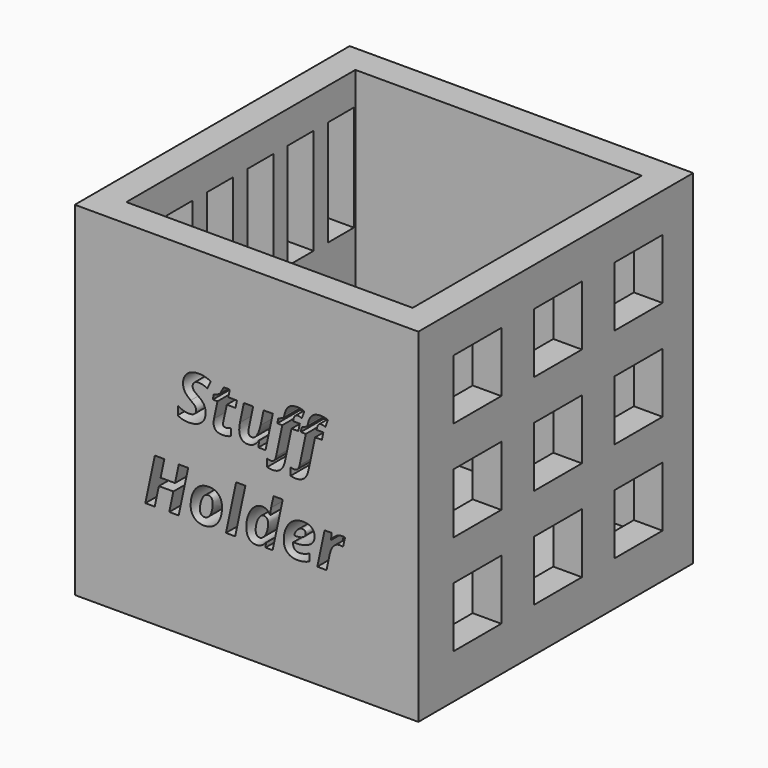
from build123d import *

# Parameters (mm, degrees)
F0_W         = 60
F0_H         = 60
F1_DEPTH     = 60
F2_W         = 50
F2_H         = 50
F3_DEPTH     = 55
F4_TEXT_SIZE = 11.0161878789
F5_DEPTH     = 10
F6_W         = 10.4811163619
F6_H         = 10.4811154306
F7_DEPTH     = 10
F8_W         = 5.6469417632
F8_H         = 18.4732027113
F9_DEPTH     = 10


# Not quite as in the source:
# - Text() gives the source's letters only with a copy of the font that has no kerning and outlines rounded to 1/6400 em; it was checked with that copy


with BuildPart() as f1:
    # F0 (on Right) → F1 (new body)
    with BuildSketch(Plane.YZ):
        with Locations((0.1416392624, -0.4152884824)):
            Rectangle(F0_W, F0_H)
    extrude(amount=F1_DEPTH)

    # F2 (on face) → F3 (cut)
    with BuildSketch(Plane.XY.offset(29.5847115176)):
        with Locations((30, 0.1416392624)):
            Rectangle(F2_W, F2_H)
    extrude(amount=-F3_DEPTH, mode=Mode.SUBTRACT)

    # F4 (on face) → F5 (cut)
    with BuildSketch(Plane.XZ.offset(29.8583607376)):
        with Locations((17.7640982414, 2.6910963934)):
            Text('Stuff', F4_TEXT_SIZE, font='Open Sans', font_style=FontStyle.BOLDITALIC, text_align=(TextAlign.LEFT, TextAlign.BOTTOM))
        with Locations((12.039123103, -12.290919122)):
            Text('Holder', F4_TEXT_SIZE, font='Open Sans', font_style=FontStyle.BOLDITALIC, text_align=(TextAlign.LEFT, TextAlign.BOTTOM))
    extrude(amount=-F5_DEPTH, mode=Mode.SUBTRACT)

    # F6 (on face) → F7 (cut)
    with BuildSketch(Plane.YZ.offset(60)):
        with Locations((-16.9964036904, 17.56295003)):
            Rectangle(F6_W, F6_H)
        with Locations((-16.9964036904, 0.06295003)):
            Rectangle(F6_W, F6_H)
        with Locations((-16.9964036904, -17.43704997)):
            Rectangle(F6_W, F6_H)
        with Locations((0.6035963096, 17.56295003)):
            Rectangle(F6_W, F6_H)
        with Locations((0.6035963096, 0.06295003)):
            Rectangle(F6_W, F6_H)
        with Locations((0.6035963096, -17.43704997)):
            Rectangle(F6_W, F6_H)
        with Locations((18.2035963096, 17.56295003)):
            Rectangle(F6_W, F6_H)
        with Locations((18.2035963096, 0.06295003)):
            Rectangle(F6_W, F6_H)
        with Locations((18.2035963096, -17.43704997)):
            Rectangle(F6_W, F6_H)
    extrude(amount=-F7_DEPTH, mode=Mode.SUBTRACT)

    # F8 (on face) → F9 (cut)
    with BuildSketch(Plane(origin=(0, 0, 0), x_dir=(0, -1, 0), z_dir=(-1, 0, 0))):
        with Locations((-22, 14.7)):
            Rectangle(F8_W, F8_H)
        with Locations((-22, -14.7)):
            Rectangle(F8_W, F8_H)
        with Locations((-13.2, 14.7)):
            Rectangle(F8_W, F8_H)
        with Locations((-13.2, -14.7)):
            Rectangle(F8_W, F8_H)
        with Locations((-4.4, 14.7)):
            Rectangle(F8_W, F8_H)
        with Locations((-4.4, -14.7)):
            Rectangle(F8_W, F8_H)
        with Locations((4.4, 14.7)):
            Rectangle(F8_W, F8_H)
        with Locations((4.4, -14.7)):
            Rectangle(F8_W, F8_H)
        with Locations((13.2, 14.7)):
            Rectangle(F8_W, F8_H)
        with Locations((13.2, -14.7)):
            Rectangle(F8_W, F8_H)
        with Locations((22, 14.7)):
            Rectangle(F8_W, F8_H)
        with Locations((22, -14.7)):
            Rectangle(F8_W, F8_H)
    extrude(amount=-F9_DEPTH, mode=Mode.SUBTRACT)


solid = f1.part
